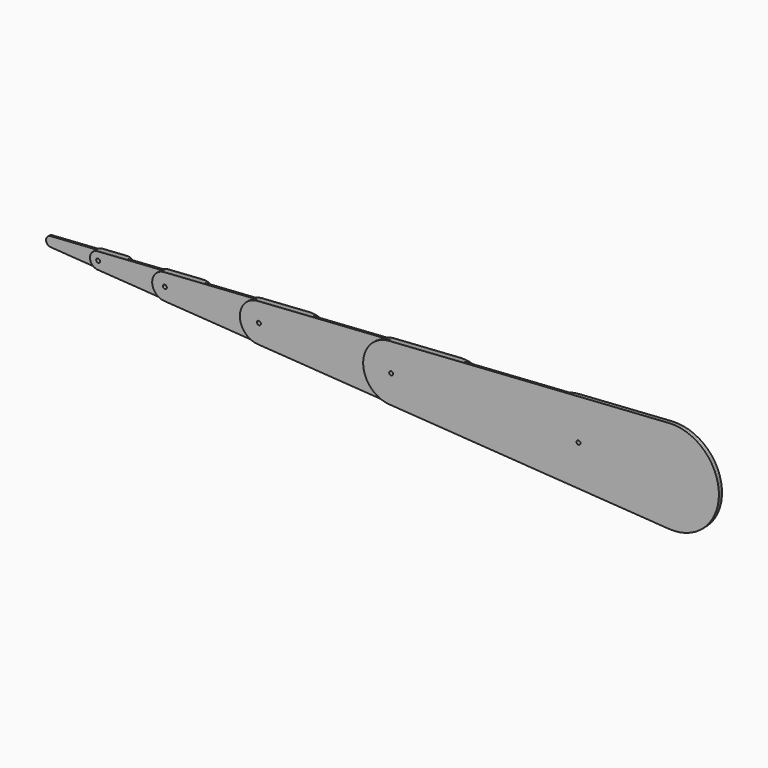
from build123d import *

# Parameters (mm, degrees)
F0_R      = 4
F1_DEPTH  = 4
F2_R      = 4
F3_DEPTH  = 4
F4_R      = 4
F5_DEPTH  = 4
F6_R      = 4
F7_DEPTH  = 4
F8_R      = 4
F9_DEPTH  = 4
F10_R     = 4
F11_DEPTH = 4
F12_R     = 4
F13_DEPTH = 4
F14_R     = 4
F15_DEPTH = 4
F16_R     = 4
F17_DEPTH = 4
F18_R     = 4
F19_DEPTH = 4


with BuildPart() as f1:
    # F0 (on Front) → F1 (new body)
    with BuildSketch(Plane.XZ):
        with BuildLine():
            ThreePointArc((12.3308842136, 16.7760425446), (-6.335782453, 36.7315486073), (12.3308842136, 56.6870546701))
            Line((12.3308842136, 56.6870546701), (-137.0024491197, 46.7093016387))
            ThreePointArc((-137.0024491197, 46.7093016387), (-129.5044819424, 44.0345160408), (-126.335782453, 36.7315486073))
            ThreePointArc((-126.335782453, 36.7315486073), (-129.5044819424, 29.4285811739), (-137.0024491197, 26.753795576))
            Line((-137.0024491197, 26.753795576), (12.3308842136, 16.7760425446))
        make_face()
        with Locations((-36.335782453, 36.7315486073)):
            Circle(F0_R, mode=Mode.SUBTRACT)
        with BuildLine():
            ThreePointArc((-126.335782453, 36.7315486073), (-129.5044819424, 44.0345160408), (-137.0024491197, 46.7093016387))
            ThreePointArc((-137.0024491197, 46.7093016387), (-146.335782453, 36.7315486073), (-137.0024491197, 26.753795576))
            ThreePointArc((-137.0024491197, 26.753795576), (-129.5044819424, 29.4285811739), (-126.335782453, 36.7315486073))
        make_face()
        with BuildLine():
            ThreePointArc((12.3308842136, 16.7760425446), (27.3268185682, 22.1256137405), (33.664217547, 36.7315486073))
            ThreePointArc((33.664217547, 36.7315486073), (27.3268185682, 51.3374834742), (12.3308842136, 56.6870546701))
            ThreePointArc((12.3308842136, 56.6870546701), (-6.335782453, 36.7315486073), (12.3308842136, 16.7760425446))
        make_face()
    extrude(amount=F1_DEPTH)


with BuildPart() as f3:
    # F2 (on face) → F3 (new body)
    with BuildSketch(Plane(origin=(0, 0, 0), x_dir=(-1, 0, 0), z_dir=(0, 1, 0))):
        with BuildLine():
            ThreePointArc((22.7091269114, 27.1350890244), (29.1576254272, 21.6898785042), (37.4468935642, 20.1019602217))
            ThreePointArc((37.4468935642, 20.1019602217), (48.507394842, 25.3460477563), (53.0024491197, 36.7315486073))
            ThreePointArc((53.0024491197, 36.7315486073), (48.507394842, 48.1170494584), (37.4468935642, 53.361136993))
            ThreePointArc((37.4468935642, 53.361136993), (29.1576254272, 51.7732187105), (22.7091269114, 46.3280081903))
            ThreePointArc((22.7091269114, 46.3280081903), (19.6691157864, 36.7315486073), (22.7091269114, 27.1350890244))
        make_face()
        with Locations((36.335782453, 36.7315486073)):
            Circle(F2_R, mode=Mode.SUBTRACT)
        with BuildLine():
            Line((-12.3308842136, 16.7760425446), (37.4468935642, 20.1019602217))
            ThreePointArc((37.4468935642, 20.1019602217), (29.1576254272, 21.6898785042), (22.7091269114, 27.1350890244))
            Line((22.7091269114, 27.1350890244), (-12.864217547, 24.7582449697))
            ThreePointArc((-12.864217547, 24.7582449697), (-25.664217547, 36.7315486073), (-12.864217547, 48.704852245))
            Line((-12.864217547, 48.704852245), (22.7091269114, 46.3280081903))
            ThreePointArc((22.7091269114, 46.3280081903), (29.1576254272, 51.7732187105), (37.4468935642, 53.361136993))
            Line((37.4468935642, 53.361136993), (-12.3308842136, 56.6870546701))
            ThreePointArc((-12.3308842136, 56.6870546701), (-33.664217547, 36.7315486073), (-12.3308842136, 16.7760425446))
        make_face()
    extrude(amount=F3_DEPTH)


with BuildPart() as f5:
    # F4 (on face) → F5 (new body)
    with BuildSketch(Plane.XZ.offset(4)):
        with BuildLine():
            ThreePointArc((-37.4468935642, 20.1019602217), (-24.950281602, 24.5599362183), (-19.6691157864, 36.7315486073))
            ThreePointArc((-19.6691157864, 36.7315486073), (-24.950281602, 48.9031609964), (-37.4468935642, 53.361136993))
            ThreePointArc((-37.4468935642, 53.361136993), (-53.0024491197, 36.7315486073), (-37.4468935642, 20.1019602217))
        make_face()
        with Locations((-36.335782453, 36.7315486073)):
            Circle(F4_R, mode=Mode.SUBTRACT)
        with BuildLine():
            Line((171.6197731025, 67.329991237), (12.3308842136, 56.6870546701))
            ThreePointArc((12.3308842136, 56.6870546701), (33.664217547, 36.7315486073), (12.3308842136, 16.7760425446))
            Line((12.3308842136, 16.7760425446), (171.6197731025, 6.1331059777))
            ThreePointArc((171.6197731025, 6.1331059777), (142.9975508803, 36.7315486073), (171.6197731025, 67.329991237))
        make_face()
        with Locations((103.664217547, 36.7315486073)):
            Circle(F4_R, mode=Mode.SUBTRACT)
        with BuildLine():
            ThreePointArc((-37.4468935642, 53.361136993), (-24.950281602, 48.9031609964), (-19.6691157864, 36.7315486073))
            ThreePointArc((-19.6691157864, 36.7315486073), (-24.950281602, 24.5599362183), (-37.4468935642, 20.1019602217))
            Line((-37.4468935642, 20.1019602217), (12.3308842136, 16.7760425446))
            ThreePointArc((12.3308842136, 16.7760425446), (33.664217547, 36.7315486073), (12.3308842136, 56.6870546701))
            Line((12.3308842136, 56.6870546701), (-37.4468935642, 53.361136993))
        make_face()
        with BuildLine():
            ThreePointArc((204.3308842136, 36.7315486073), (194.6135391129, 59.1273154031), (171.6197731025, 67.329991237))
            ThreePointArc((171.6197731025, 67.329991237), (142.9975508803, 36.7315486073), (171.6197731025, 6.1331059777))
            ThreePointArc((171.6197731025, 6.1331059777), (194.6135391129, 14.3357818116), (204.3308842136, 36.7315486073))
        make_face()
    extrude(amount=F5_DEPTH)


with BuildPart() as f7:
    # F6 (on face) → F7 (new body)
    with BuildSketch(Plane(origin=(0, -4, 0), x_dir=(-1, 0, 0), z_dir=(0, 1, 0))):
        with BuildLine():
            ThreePointArc((-101.9308842136, 10.7893907257), (-84.6765022201, 18.9701672797), (-77.664217547, 36.7315486073))
            ThreePointArc((-77.664217547, 36.7315486073), (-84.6765022201, 54.492929935), (-101.9308842136, 62.673706489))
            ThreePointArc((-101.9308842136, 62.673706489), (-114.1684948062, 60.5151597558), (-124.0066171202, 52.9237312768))
            ThreePointArc((-124.0066171202, 52.9237312768), (-129.664217547, 36.7315486073), (-124.0066171202, 20.5393659379))
            ThreePointArc((-124.0066171202, 20.5393659379), (-114.1684948062, 12.9479374589), (-101.9308842136, 10.7893907257))
        make_face()
        with Locations((-103.664217547, 36.7315486073)):
            Circle(F6_R, mode=Mode.SUBTRACT)
        with BuildLine():
            ThreePointArc((-124.0066171202, 52.9237312768), (-114.1684948062, 60.5151597558), (-101.9308842136, 62.673706489))
            Line((-101.9308842136, 62.673706489), (-171.6197731025, 67.329991237))
            ThreePointArc((-171.6197731025, 67.329991237), (-204.3308842136, 36.7315486073), (-171.6197731025, 6.1331059777))
            Line((-171.6197731025, 6.1331059777), (-101.9308842136, 10.7893907257))
            ThreePointArc((-101.9308842136, 10.7893907257), (-114.1684948062, 12.9479374589), (-124.0066171202, 20.5393659379))
            Line((-124.0066171202, 20.5393659379), (-172.3664397692, 17.3081893729))
            ThreePointArc((-172.3664397692, 17.3081893729), (-193.1308842136, 36.7315486073), (-172.3664397692, 56.1549078418))
            Line((-172.3664397692, 56.1549078418), (-124.0066171202, 52.9237312768))
        make_face()
    extrude(amount=F7_DEPTH)


with BuildPart() as f9:
    # F8 (on face) → F9 (new body)
    with BuildSketch(Plane.XZ.offset(8)):
        with BuildLine():
            ThreePointArc((101.9308842136, 10.7893907257), (121.4255988746, 17.7438332805), (129.664217547, 36.7315486073))
            ThreePointArc((129.664217547, 36.7315486073), (121.4255988746, 55.7192639342), (101.9308842136, 62.673706489))
            ThreePointArc((101.9308842136, 62.673706489), (77.664217547, 36.7315486073), (101.9308842136, 10.7893907257))
        make_face()
        with Locations((103.664217547, 36.7315486073)):
            Circle(F8_R, mode=Mode.SUBTRACT)
        with BuildLine():
            ThreePointArc((101.9308842136, 62.673706489), (121.4255988746, 55.7192639342), (129.664217547, 36.7315486073))
            ThreePointArc((129.664217547, 36.7315486073), (121.4255988746, 17.7438332805), (101.9308842136, 10.7893907257))
            Line((101.9308842136, 10.7893907257), (171.6197731025, 6.1331059777))
            ThreePointArc((171.6197731025, 6.1331059777), (204.3308842136, 36.7315486073), (171.6197731025, 67.329991237))
            Line((171.6197731025, 67.329991237), (101.9308842136, 62.673706489))
        make_face()
        with BuildLine():
            Line((394.624217547, 82.2301024305), (171.6197731025, 67.329991237))
            ThreePointArc((171.6197731025, 67.329991237), (204.3308842136, 36.7315486073), (171.6197731025, 6.1331059777))
            Line((171.6197731025, 6.1331059777), (394.624217547, -8.7670052158))
            ThreePointArc((394.624217547, -8.7670052158), (352.064217547, 36.7315486073), (394.624217547, 82.2301024305))
        make_face()
        with Locations((299.664217547, 36.7315486073)):
            Circle(F8_R, mode=Mode.SUBTRACT)
        with BuildLine():
            ThreePointArc((443.264217547, 36.7315486073), (428.8149478755, 70.0330801037), (394.624217547, 82.2301024305))
            ThreePointArc((394.624217547, 82.2301024305), (352.064217547, 36.7315486073), (394.624217547, -8.7670052158))
            ThreePointArc((394.624217547, -8.7670052158), (428.8149478755, 3.430017111), (443.264217547, 36.7315486073))
        make_face()
    extrude(amount=F9_DEPTH)


with BuildPart() as f11:
    # F10 (on face) → F11 (new body)
    with BuildSketch(Plane(origin=(0, -8, 0), x_dir=(-1, 0, 0), z_dir=(0, 1, 0))):
        with BuildLine():
            ThreePointArc((-297.0597731025, -2.2482065686), (-271.1339581071, 10.0439346125), (-260.5975508803, 36.7315486073))
            ThreePointArc((-260.5975508803, 36.7315486073), (-271.1339581071, 63.4191626022), (-297.0597731025, 75.7113037833))
            ThreePointArc((-297.0597731025, 75.7113037833), (-314.7977246755, 72.7479532924), (-329.328750734, 62.1524045182))
            ThreePointArc((-329.328750734, 62.1524045182), (-338.7308842136, 36.7315486073), (-329.328750734, 11.3106926965))
            ThreePointArc((-329.328750734, 11.3106926965), (-314.7977246755, 0.7151439223), (-297.0597731025, -2.2482065686))
        make_face()
        with Locations((-299.664217547, 36.7315486073)):
            Circle(F10_R, mode=Mode.SUBTRACT)
        with BuildLine():
            ThreePointArc((-329.328750734, 62.1524045182), (-314.7977246755, 72.7479532924), (-297.0597731025, 75.7113037833))
            Line((-297.0597731025, 75.7113037833), (-394.624217547, 82.2301024305))
            ThreePointArc((-394.624217547, 82.2301024305), (-443.264217547, 36.7315486073), (-394.624217547, -8.7670052158))
            Line((-394.624217547, -8.7670052158), (-297.0597731025, -2.2482065686))
            ThreePointArc((-297.0597731025, -2.2482065686), (-314.7977246755, 0.7151439223), (-329.328750734, 11.3106926965))
            Line((-329.328750734, 11.3106926965), (-395.6695508803, 6.8781115374))
            ThreePointArc((-395.6695508803, 6.8781115374), (-427.584217547, 36.7315486073), (-395.6695508803, 66.5849856773))
            Line((-395.6695508803, 66.5849856773), (-329.328750734, 62.1524045182))
        make_face()
    extrude(amount=F11_DEPTH)


with BuildPart() as f13:
    # F12 (on face) → F13 (new body)
    with BuildSketch(Plane.XZ.offset(12)):
        with BuildLine():
            ThreePointArc((297.0597731025, -2.2482065686), (326.3518315419, 8.2012891675), (338.7308842136, 36.7315486073))
            ThreePointArc((338.7308842136, 36.7315486073), (326.3518315419, 65.2618080472), (297.0597731025, 75.7113037833))
            ThreePointArc((297.0597731025, 75.7113037833), (260.5975508803, 36.7315486073), (297.0597731025, -2.2482065686))
        make_face()
        with Locations((299.664217547, 36.7315486073)):
            Circle(F12_R, mode=Mode.SUBTRACT)
        with BuildLine():
            ThreePointArc((297.0597731025, 75.7113037833), (326.3518315419, 65.2618080472), (338.7308842136, 36.7315486073))
            ThreePointArc((338.7308842136, 36.7315486073), (326.3518315419, 8.2012891675), (297.0597731025, -2.2482065686))
            Line((297.0597731025, -2.2482065686), (394.624217547, -8.7670052158))
            ThreePointArc((394.624217547, -8.7670052158), (443.264217547, 36.7315486073), (394.624217547, 82.2301024305))
            Line((394.624217547, 82.2301024305), (297.0597731025, 75.7113037833))
        make_face()
        with BuildLine():
            Line((706.8304397692, 103.0902581015), (394.624217547, 82.2301024305))
            ThreePointArc((394.624217547, 82.2301024305), (443.264217547, 36.7315486073), (394.624217547, -8.7670052158))
            Line((394.624217547, -8.7670052158), (706.8304397692, -29.6271608868))
            ThreePointArc((706.8304397692, -29.6271608868), (644.7575508803, 36.7315486073), (706.8304397692, 103.0902581015))
        make_face()
        with Locations((574.064217547, 36.7315486073)):
            Circle(F12_R, mode=Mode.SUBTRACT)
        with BuildLine():
            ThreePointArc((777.7708842136, 36.7315486073), (756.6969201431, 85.3011506844), (706.8304397692, 103.0902581015))
            ThreePointArc((706.8304397692, 103.0902581015), (644.7575508803, 36.7315486073), (706.8304397692, -29.6271608868))
            ThreePointArc((706.8304397692, -29.6271608868), (756.6969201431, -11.8380534697), (777.7708842136, 36.7315486073))
        make_face()
    extrude(amount=F13_DEPTH)


with BuildPart() as f15:
    # F14 (on face) → F15 (new body)
    with BuildSketch(Plane(origin=(0, -12, 0), x_dir=(-1, 0, 0), z_dir=(0, 1, 0))):
        with BuildLine():
            ThreePointArc((-570.240217547, -20.5008427807), (-532.174396349, -2.4527911217), (-516.704217547, 36.7315486073))
            ThreePointArc((-516.704217547, 36.7315486073), (-532.174396349, 75.9158883364), (-570.240217547, 93.9639399954))
            ThreePointArc((-570.240217547, 93.9639399954), (-595.6611715973, 89.8704343291), (-616.7302572302, 75.0692409968))
            ThreePointArc((-616.7302572302, 75.0692409968), (-631.424217547, 36.7315486073), (-616.7302572302, -1.6061437821))
            ThreePointArc((-616.7302572302, -1.6061437821), (-595.6611715973, -16.4073371144), (-570.240217547, -20.5008427807))
        make_face()
        with Locations((-574.064217547, 36.7315486073)):
            Circle(F14_R, mode=Mode.SUBTRACT)
        with BuildLine():
            ThreePointArc((-616.7302572302, 75.0692409968), (-595.6611715973, 89.8704343291), (-570.240217547, 93.9639399954))
            Line((-570.240217547, 93.9639399954), (-706.8304397692, 103.0902581015))
            ThreePointArc((-706.8304397692, 103.0902581015), (-777.7708842136, 36.7315486073), (-706.8304397692, -29.6271608868))
            Line((-706.8304397692, -29.6271608868), (-570.240217547, -20.5008427807))
            ThreePointArc((-570.240217547, -20.5008427807), (-595.6611715973, -16.4073371144), (-616.7302572302, -1.6061437821))
            Line((-616.7302572302, -1.6061437821), (-708.2939064358, -7.7239974323))
            ThreePointArc((-708.2939064358, -7.7239974323), (-755.8188842136, 36.7315486073), (-708.2939064358, 81.187094647))
            Line((-708.2939064358, 81.187094647), (-616.7302572302, 75.0692409968))
        make_face()
    extrude(amount=F15_DEPTH)


with BuildPart() as f17:
    # F16 (on face) → F17 (new body)
    with BuildSketch(Plane.XZ.offset(16)):
        with BuildLine():
            ThreePointArc((570.240217547, -20.5008427807), (613.248557276, -5.1582725906), (631.424217547, 36.7315486073))
            ThreePointArc((631.424217547, 36.7315486073), (613.248557276, 78.6213698053), (570.240217547, 93.9639399954))
            ThreePointArc((570.240217547, 93.9639399954), (516.704217547, 36.7315486073), (570.240217547, -20.5008427807))
        make_face()
        with Locations((574.064217547, 36.7315486073)):
            Circle(F16_R, mode=Mode.SUBTRACT)
        with BuildLine():
            ThreePointArc((570.240217547, 93.9639399954), (613.248557276, 78.6213698053), (631.424217547, 36.7315486073))
            ThreePointArc((631.424217547, 36.7315486073), (613.248557276, -5.1582725906), (570.240217547, -20.5008427807))
            Line((570.240217547, -20.5008427807), (706.8304397692, -29.6271608868))
            ThreePointArc((706.8304397692, -29.6271608868), (777.7708842136, 36.7315486073), (706.8304397692, 103.0902581015))
            Line((706.8304397692, 103.0902581015), (570.240217547, 93.9639399954))
        make_face()
        with BuildLine():
            Line((1143.9191508803, 132.2944760409), (706.8304397692, 103.0902581015))
            ThreePointArc((706.8304397692, 103.0902581015), (777.7708842136, 36.7315486073), (706.8304397692, -29.6271608868))
            Line((706.8304397692, -29.6271608868), (1143.9191508803, -58.8313788262))
            ThreePointArc((1143.9191508803, -58.8313788262), (1054.528217547, 36.7315486073), (1143.9191508803, 132.2944760409))
        make_face()
        with Locations((958.224217547, 36.7315486073)):
            Circle(F16_R, mode=Mode.SUBTRACT)
        with BuildLine():
            ThreePointArc((1246.080217547, 36.7315486073), (1215.7316813177, 106.6764494975), (1143.9191508803, 132.2944760409))
            ThreePointArc((1143.9191508803, 132.2944760409), (1054.528217547, 36.7315486073), (1143.9191508803, -58.8313788262))
            ThreePointArc((1143.9191508803, -58.8313788262), (1215.7316813177, -33.2133522828), (1246.080217547, 36.7315486073))
        make_face()
    extrude(amount=F17_DEPTH)


with BuildPart() as f19:
    # F18 (on face) → F19 (new body)
    with BuildSketch(Plane(origin=(0, -16, 0), x_dir=(-1, 0, 0), z_dir=(0, 1, 0))):
        with BuildLine():
            ThreePointArc((-952.6928397692, -46.0545334777), (-897.6310098875, -19.9482071495), (-875.2535508803, 36.7315486073))
            ThreePointArc((-875.2535508803, 36.7315486073), (-897.6310098875, 93.4113043642), (-952.6928397692, 119.5176306924))
            ThreePointArc((-952.6928397692, 119.5176306924), (-988.8584096054, 113.8397699851), (-1019.0601869407, 93.1506619913))
            ThreePointArc((-1019.0601869407, 93.1506619913), (-1041.1948842136, 36.7315486073), (-1019.0601869407, -19.6875647766))
            ThreePointArc((-1019.0601869407, -19.6875647766), (-988.8584096054, -40.3766727704), (-952.6928397692, -46.0545334777))
        make_face()
        with Locations((-958.224217547, 36.7315486073)):
            Circle(F18_R, mode=Mode.SUBTRACT)
        with BuildLine():
            ThreePointArc((-1019.0601869407, 93.1506619913), (-988.8584096054, 113.8397699851), (-952.6928397692, 119.5176306924))
            Line((-952.6928397692, 119.5176306924), (-1143.9191508803, 132.2944760409))
            ThreePointArc((-1143.9191508803, 132.2944760409), (-1246.080217547, 36.7315486073), (-1143.9191508803, -58.8313788262))
            Line((-1143.9191508803, -58.8313788262), (-952.6928397692, -46.0545334777))
            ThreePointArc((-952.6928397692, -46.0545334777), (-988.8584096054, -40.3766727704), (-1019.0601869407, -19.6875647766))
            Line((-1019.0601869407, -19.6875647766), (-1145.9680042136, -28.1669499898))
            ThreePointArc((-1145.9680042136, -28.1669499898), (-1215.347417547, 36.7315486073), (-1145.9680042136, 101.6300472045))
            Line((-1145.9680042136, 101.6300472045), (-1019.0601869407, 93.1506619913))
        make_face()
    extrude(amount=F19_DEPTH)


solid = Compound([f1.part, f3.part, f5.part, f7.part, f9.part, f11.part, f13.part, f15.part, f17.part, f19.part])
